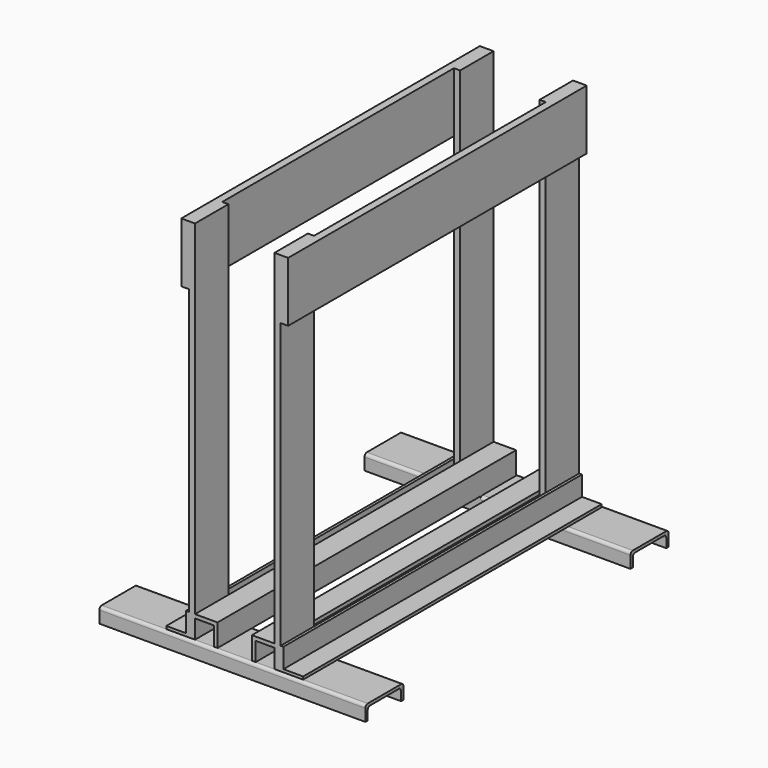
from build123d import *

# Parameters (mm, degrees)
F1_DEPTH  = 631.5
F2_DEPTH  = 70.75
F3_W      = 10.45
F3_H      = 70.75
F4_DEPTH  = 620
F5_W      = 450
F5_H      = 80.75
F6_DEPTH  = 25.4
F7_R      = 4.99999
F9_DEPTH  = 631.5
F10_DEPTH = 70.75
F11_W     = 10.45
F11_H     = 70.75
F12_DEPTH = 620
F13_W     = 12.75
F13_H     = 101.2
F14_DEPTH = 631.5
F16_DEPTH = 631.5
F18_DEPTH = 300
F19_DEPTH = 300


# Not quite as in the source:
# - a fillet or chamfer is up to 0.001 mm smaller than in the source, because OpenCascade refuses the exact size


with BuildPart() as f1:
    # F0 (on Front) → F1 (new body)
    with BuildSketch(Plane.XZ):
        Polygon((0, 38.1), (0, 31.75), (31.75, 31.75), (31.75, 0), (38.1, 0), (38.1, 38.1), align=None)
    extrude(amount=F1_DEPTH)

    # F0 (on Front) → F2 (join)
    with BuildSketch(Plane.XZ):
        Polygon((-10.45, 0), (0, 0), (0, 31.75), (0, 38.1), (0, 620), (-10.45, 620), align=None)
    extrude(amount=F2_DEPTH)

    # F3 (on Top) → F4 (join)
    with BuildSketch(Plane.XY):
        with Locations((-5.225, -596.125)):
            Rectangle(F3_W, F3_H)
    extrude(amount=F4_DEPTH)

    # F5 (on Top) → F6 (join)
    with BuildSketch(Plane.XY):
        with Locations((67.2, -35.375)):
            Rectangle(F5_W, F5_H)
        with Locations((67.2, -596.125)):
            Rectangle(F5_W, F5_H)
    extrude(amount=-F6_DEPTH)

    # F7 (radius 5 in the source; OpenCascade refuses exactly that, so slightly less here)
    f7_edges = [f1.edges().sort_by_distance(p)[0] for p in [
        (67.2, -636.5, 0),
        (165.15, -555.75, 0),
        (165.15, -75.75, 0),
        (67.2, 5, 0),
        (-63.025, -75.75, 0),
        (-63.025, -555.75, 0),
    ]]
    fillet(f7_edges, radius=F7_R)

    # F8 (on Front) → F9 (join)
    with BuildSketch(Plane.XZ):
        Polygon((102.65, 31.75), (134.4, 31.75), (134.4, 38.1), (96.3, 38.1), (96.3, 0), (102.65, 0), align=None)
    extrude(amount=F9_DEPTH)

    # F8 (on Front) → F10 (join)
    with BuildSketch(Plane.XZ):
        Polygon((134.4, 31.75), (134.4, 0), (144.85, 0), (144.85, 620), (134.4, 620), (134.4, 38.1), align=None)
        Polygon((102.65, 31.75), (134.4, 31.75), (134.4, 38.1), (96.3, 38.1), (96.3, 0), (102.65, 0), align=None)
    extrude(amount=F10_DEPTH)

    # F11 (on Top) → F12 (join)
    with BuildSketch(Plane.XY):
        with Locations((139.625, -596.125)):
            Rectangle(F11_W, F11_H)
    extrude(amount=F12_DEPTH)

    # F13 (on Front) → F14 (join)
    with BuildSketch(Plane.XZ):
        with Locations((-16.825, 569.4)):
            Rectangle(F13_W, F13_H)
        with Locations((151.225, 569.4)):
            Rectangle(F13_W, F13_H)
    extrude(amount=F14_DEPTH)

    # F15 (on Front) → F16 (join)
    with BuildSketch(Plane.XZ):
        Polygon((-48.55, 4.763), (-48.55, 0), (-10.45, 0), (-10.45, 38.1), (-15.213, 38.1), (-15.213, 4.763), align=None)
        Polygon((144.85, 0), (182.95, 0), (182.95, 4.763), (149.613, 4.763), (149.613, 38.1), (144.85, 38.1), align=None)
    extrude(amount=F16_DEPTH)

    # F17 (on Right) → F18 (cut)
    with BuildSketch(Plane.YZ):
        with BuildLine():
            Line((-631.5, -10), (-631.5, -25.4))
            Line((-631.5, -25.4), (-560.75, -25.4))
            Line((-560.75, -25.4), (-560.75, -10))
            ThreePointArc((-560.75, -10), (-562.2144660941, -6.4644660941), (-565.75, -5))
            Line((-565.75, -5), (-626.5, -5))
            ThreePointArc((-626.5, -5), (-630.0355339059, -6.4644660941), (-631.5, -10))
        make_face()
        with BuildLine():
            Line((-5, -5), (-65.75, -5))
            ThreePointArc((-65.75, -5), (-69.2855339059, -6.4644660941), (-70.75, -10))
            Line((-70.75, -10), (-70.75, -25.4))
            Line((-70.75, -25.4), (0, -25.4))
            Line((0, -25.4), (0, -10))
            ThreePointArc((0, -10), (-1.4644660941, -6.4644660941), (-5, -5))
        make_face()
    extrude(amount=F18_DEPTH, mode=Mode.SUBTRACT)

    # F17 (on Right) → F19 (cut)
    with BuildSketch(Plane.YZ):
        with BuildLine():
            Line((-631.5, -10), (-631.5, -25.4))
            Line((-631.5, -25.4), (-560.75, -25.4))
            Line((-560.75, -25.4), (-560.75, -10))
            ThreePointArc((-560.75, -10), (-562.2144660941, -6.4644660941), (-565.75, -5))
            Line((-565.75, -5), (-626.5, -5))
            ThreePointArc((-626.5, -5), (-630.0355339059, -6.4644660941), (-631.5, -10))
        make_face()
        with BuildLine():
            Line((-5, -5), (-65.75, -5))
            ThreePointArc((-65.75, -5), (-69.2855339059, -6.4644660941), (-70.75, -10))
            Line((-70.75, -10), (-70.75, -25.4))
            Line((-70.75, -25.4), (0, -25.4))
            Line((0, -25.4), (0, -10))
            ThreePointArc((0, -10), (-1.4644660941, -6.4644660941), (-5, -5))
        make_face()
    extrude(amount=-F19_DEPTH, mode=Mode.SUBTRACT)


solid = f1.part
